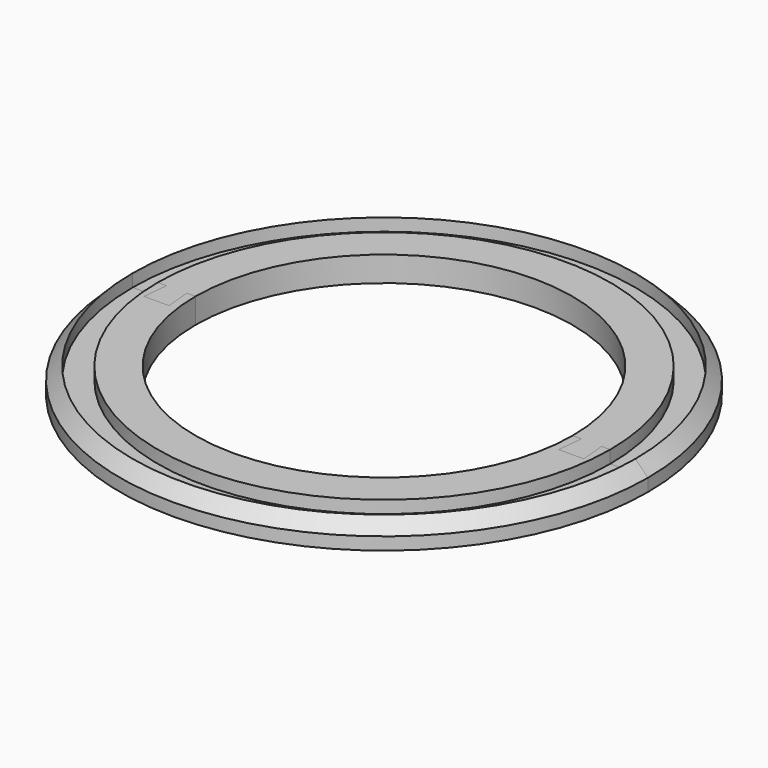
from build123d import *

# Parameters (mm, degrees)
F1_DEPTH  = 2
F2_DEPTH  = 1
F3_DEPTH  = 2
F4_DEPTH  = 2
F5_DEPTH  = 1
F6_DEPTH  = 2
F7_SIZE   = 0.99999
F7_2_SIZE = 0.99999


# Not quite as in the source:
# - a fillet or chamfer is up to 0.001 mm smaller than in the source, because OpenCascade refuses the exact size


with BuildPart() as f1:
    # F0 (on Top) → F1 (new body)
    with BuildSketch(Plane.XY):
        with BuildLine():
            Line((20, 0), (21, 0))
            ThreePointArc((21, 0), (0, 21), (-21, 0))
            Line((-21, 0), (-20, 0))
            ThreePointArc((-20, 0), (0, 20), (20, 0))
        make_face()
    extrude(amount=F1_DEPTH)

    # F0 (on Top) → F2 (join)
    with BuildSketch(Plane.XY):
        with BuildLine():
            Line((18, 0), (20, 0))
            ThreePointArc((20, 0), (0, 20), (-20, 0))
            Line((-20, 0), (-18, 0))
            ThreePointArc((-18, 0), (0, 18), (18, 0))
        make_face()
    extrude(amount=F2_DEPTH)

    # F0 (on Top) → F3 (join)
    with BuildSketch(Plane.XY):
        with BuildLine():
            Line((17.3, 0), (18, 0))
            ThreePointArc((18, 0), (0, 18), (-18, 0))
            Line((-18, 0), (-17.3, 0))
            Line((-17.3, 0), (-17.5, -2))
            Line((-17.5, -2), (-16.5, -2))
            Line((-16.5, -2), (-15.5, -2))
            Line((-15.5, -2), (-15.7, 0))
            Line((-15.7, 0), (-15, 0))
            ThreePointArc((-15, 0), (0, 15), (15, 0))
            Line((15, 0), (15.7, 0))
            Line((15.7, 0), (15.5, -2))
            Line((15.5, -2), (16.5, -2))
            Line((16.5, -2), (17.5, -2))
            Line((17.5, -2), (17.3, 0))
        make_face()
    extrude(amount=F3_DEPTH)

    # F7 (size 1 in the source; OpenCascade refuses exactly that, so slightly less here)
    f7_edges = [f1.edges().sort_by_distance(p)[0] for p in [
        (0, 21, 2),
    ]]
    chamfer(f7_edges, length=F7_SIZE)


with BuildPart() as f4:
    # F0 (on Top) → F4 (new body)
    with BuildSketch(Plane.XY):
        with BuildLine():
            ThreePointArc((-18, 0), (0, -18), (18, 0))
            Line((18, 0), (17.3, 0))
            Line((17.3, 0), (17.5, -2))
            Line((17.5, -2), (16.5, -2))
            Line((16.5, -2), (15.5, -2))
            Line((15.5, -2), (15.7, 0))
            Line((15.7, 0), (15, 0))
            ThreePointArc((15, 0), (0, -15), (-15, 0))
            Line((-15, 0), (-15.7, 0))
            Line((-15.7, 0), (-15.5, -2))
            Line((-15.5, -2), (-16.5, -2))
            Line((-16.5, -2), (-17.5, -2))
            Line((-17.5, -2), (-17.3, 0))
            Line((-17.3, 0), (-18, 0))
        make_face()
    extrude(amount=F4_DEPTH)

    # F0 (on Top) → F5 (join)
    with BuildSketch(Plane.XY):
        with BuildLine():
            ThreePointArc((-20, 0), (0, -20), (20, 0))
            Line((20, 0), (18, 0))
            ThreePointArc((18, 0), (0, -18), (-18, 0))
            Line((-18, 0), (-20, 0))
        make_face()
    extrude(amount=F5_DEPTH)

    # F0 (on Top) → F6 (join)
    with BuildSketch(Plane.XY):
        with BuildLine():
            ThreePointArc((-21, 0), (0, -21), (21, 0))
            Line((21, 0), (20, 0))
            ThreePointArc((20, 0), (0, -20), (-20, 0))
            Line((-20, 0), (-21, 0))
        make_face()
    extrude(amount=F6_DEPTH)

    # F7#2 (size 1 in the source; OpenCascade refuses exactly that, so slightly less here)
    f7_2_edges = [f4.edges().sort_by_distance(p)[0] for p in [
        (0, -21, 2),
    ]]
    chamfer(f7_2_edges, length=F7_2_SIZE)


solid = Compound([f1.part, f4.part])
